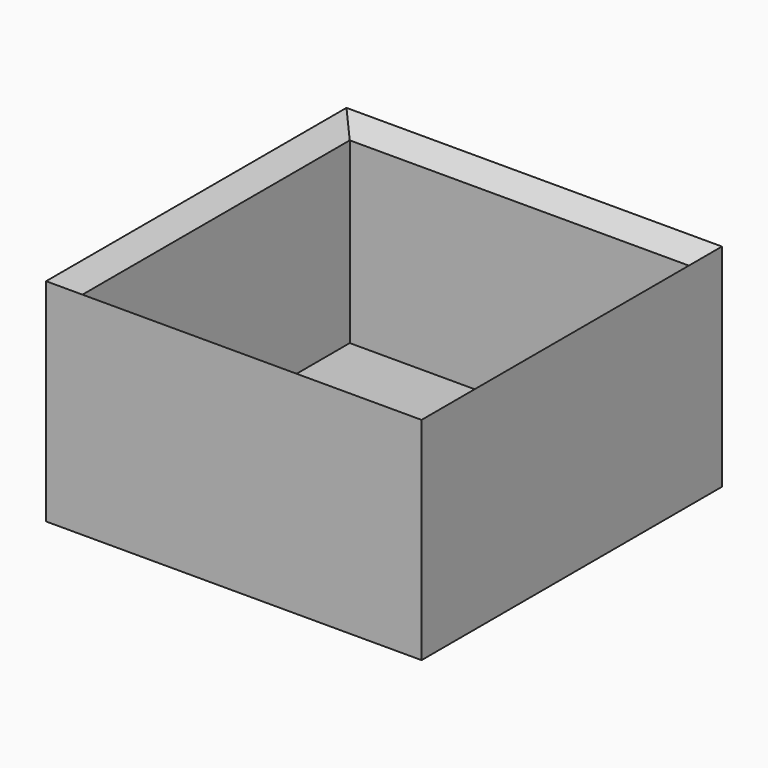
from build123d import *

# Parameters (mm, degrees)
F0_W     = 56.8
F0_H     = 56.8
F1_DEPTH = 32
F2_T     = -2.5
F3_R     = 1.5
F4_DEPTH = 2.5
F5_SIZE  = 2.49999


# Not quite as in the source:
# - a fillet or chamfer is up to 0.001 mm smaller than in the source, because OpenCascade refuses the exact size


with BuildPart() as f1:
    # F0 (on Top) → F1 (new body)
    with BuildSketch(Plane.XY):
        with Locations((28.4, 28.4)):
            Rectangle(F0_W, F0_H)
    extrude(amount=F1_DEPTH)

    # F2
    f2_openings = [f1.faces().sort_by_distance(p)[0] for p in [
        (28.4, 28.4, 32),
    ]]
    offset(amount=F2_T, openings=f2_openings)

    # F3 (on face) → F4 (cut, through all)
    with BuildSketch(Plane(origin=(0, 0, 0), x_dir=(1, 0, 0), z_dir=(0, 0, -1))):
        with Locations((25.4, -28.4)):
            Circle(F3_R)
        with Locations((31.4, -28.4)):
            Circle(F3_R)
    extrude(amount=-F4_DEPTH, mode=Mode.SUBTRACT)

    # F5 (size 2.5 in the source; OpenCascade refuses exactly that, so slightly less here)
    f5_edges = [f1.edges().sort_by_distance(p)[0] for p in [
        (2.5, 28.4, 32),
        (28.4, 2.5, 32),
        (54.3, 28.4, 32),
        (28.4, 54.3, 32),
    ]]
    chamfer(f5_edges, length=F5_SIZE)


solid = f1.part
